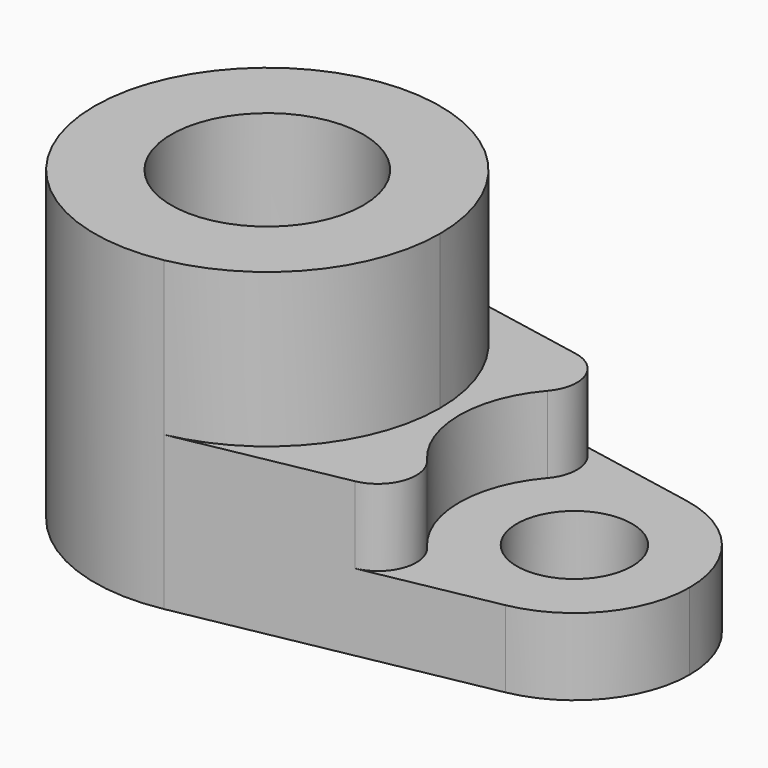
from build123d import *

# Parameters (mm, degrees)
F0_R     = 15.875
F1_DEPTH = 50.8
F2_DEPTH = 25.4
F0_R_2   = 9.525
F3_DEPTH = 12.7
F4_R     = 6.35
F4_R_2   = 6.3499


# Not quite as in the source:
# - a fillet or chamfer is up to 0.001 mm smaller than in the source, because OpenCascade refuses the exact size


with BuildPart() as f1:
    # F0 (on Top) → F1 (new body)
    with BuildSketch(Plane.XY):
        with BuildLine():
            ThreePointArc((-21.53046875, -28.0682110263), (-4.8697649831, -18.2130603251), (1.68671875, 0))
            ThreePointArc((1.68671875, 0), (-4.8697649831, 18.2130603251), (-21.53046875, 28.0682110263))
            ThreePointArc((-21.53046875, 28.0682110263), (-55.46328125, 0), (-21.53046875, -28.0682110263))
        make_face()
        with Locations((-26.88828125, 0)):
            Circle(F0_R, mode=Mode.SUBTRACT)
    extrude(amount=F1_DEPTH)

    # F0 (on Top) → F2 (join)
    with BuildSketch(Plane.XY):
        with BuildLine():
            ThreePointArc((-21.53046875, 28.0682110263), (-4.8697649831, 18.2130603251), (1.68671875, 0))
            ThreePointArc((1.68671875, 0), (-4.8697649831, -18.2130603251), (-21.53046875, -28.0682110263))
            Line((-21.53046875, -28.0682110263), (27.48359375, -18.7121406842))
            ThreePointArc((27.48359375, -18.7121406842), (4.86171875, 0), (27.48359375, 18.7121406842))
            Line((27.48359375, 18.7121406842), (-21.53046875, 28.0682110263))
        make_face()
    extrude(amount=F2_DEPTH)

    # F0 (on Top) → F3 (join)
    with BuildSketch(Plane.XY):
        with BuildLine():
            ThreePointArc((42.96171875, 0), (38.5907295946, 12.1420402167), (27.48359375, 18.7121406842))
            ThreePointArc((27.48359375, 18.7121406842), (4.86171875, 0), (27.48359375, -18.7121406842))
            ThreePointArc((27.48359375, -18.7121406842), (38.5907295946, -12.1420402167), (42.96171875, 0))
        make_face()
        with Locations((23.91171875, 0)):
            Circle(F0_R_2, mode=Mode.SUBTRACT)
    extrude(amount=F3_DEPTH)

    # F4 (call 1 of 2: OpenCascade refuses the feature's edges together)
    f4_edges = [f1.edges().sort_by_distance(p)[0] for p in [
        (27.483594, -18.712141, 6.35),
        (27.483594, -18.712141, 19.05),
    ]]
    fillet(f4_edges, radius=F4_R)

    # F4#2 (call 2 of 2) (radius 6.35 in the source; OpenCascade refuses exactly that, so slightly less here)
    f4_2_edges = [f1.edges().sort_by_distance(p)[0] for p in [
        (27.483594, 18.712141, 6.35),
        (27.483594, 18.712141, 19.05),
    ]]
    fillet(f4_2_edges, radius=F4_R_2)


solid = f1.part
